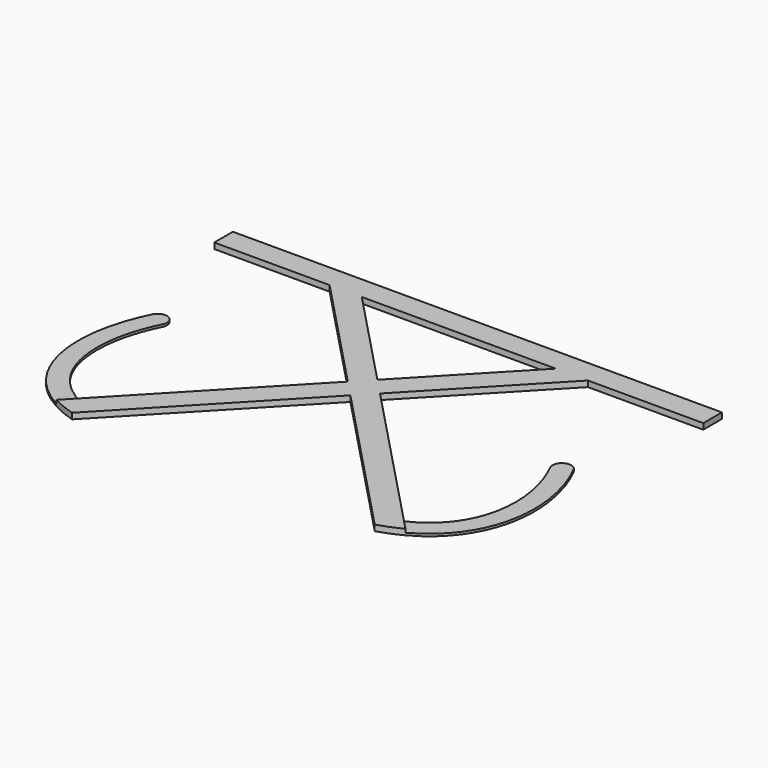
from build123d import *

# Parameters (mm, degrees)
F1_DEPTH = 2.5
F2_DEPTH = 1


with BuildPart() as f1:
    # F0 (on Top) → F1 (new body)
    with BuildSketch(Plane.XY):
        Polygon((51.1834802784, 68.1774026233), (-51.1834802784, 68.1774026233), (-41.6495295118, 58.1774026233), (41.6495295118, 58.1774026233), align=None)
        Polygon((55.4660492335, 58.1774026233), (41.6495295118, 58.1774026233), (0, 14.4919142756), (6.9082598608, 7.2459571378), align=None)
        Polygon((65, 68.1774026233), (51.1834802784, 68.1774026233), (41.6495295118, 58.1774026233), (55.4660492335, 58.1774026233), align=None)
        Polygon((105, 68.1774026233), (65, 68.1774026233), (55.4660492335, 58.1774026233), (105, 58.1774026233), align=None)
        Polygon((0, 14.4919142756), (-6.9082598608, 7.2459571378), (0, 0), (6.9082598608, 7.2459571378), align=None)
        Polygon((-41.6495295118, 58.1774026233), (-55.4660492335, 58.1774026233), (-6.9082598608, 7.2459571378), (0, 14.4919142756), align=None)
        Polygon((-65, 68.1774026233), (-105, 68.1774026233), (-105, 58.1774026233), (-55.4660492335, 58.1774026233), align=None)
        Polygon((-51.1834802784, 68.1774026233), (-65, 68.1774026233), (-55.4660492335, 58.1774026233), (-41.6495295118, 58.1774026233), align=None)
        Polygon((0, 0), (-6.9082598608, 7.2459571378), (-69.1652305646, -58.0543283665), (-72.2377126812, -61.2770029868), (-65, -68.1774026233), align=None)
        Polygon((6.9082598608, 7.2459571378), (0, 0), (65, -68.1774026233), (72.2377126812, -61.2770029868), (69.1652305646, -58.0543283665), align=None)
        with BuildLine():
            Line((72.2377126812, -61.2770029868), (65, -68.1774026233))
            add(Edge.make_bspline(
                [(65, -68.1774026233), (68.6268745658, -67.0893650818), (71.9339432438, -65.7183547634), (74.930951741, -64.1018959674)],
                knots=[0, 0, 0, 0, 8.3760284317, 8.3760284317, 8.3760284317, 8.3760284317], degree=3))
            Line((74.930951741, -64.1018959674), (72.2377126812, -61.2770029868))
        make_face()
        with BuildLine():
            add(Edge.make_bspline(
                [(-65, -68.1774026233), (-68.6268745658, -67.0893650818), (-71.9339432438, -65.7183547634), (-74.930951741, -64.1018959674)],
                knots=[0, 0, 0, 0, 8.3760284317, 8.3760284317, 8.3760284317, 8.3760284317], degree=3))
            Line((-65, -68.1774026233), (-72.2377126812, -61.2770029868))
            Line((-72.2377126812, -61.2770029868), (-74.930951741, -64.1018959674))
        make_face()
    extrude(amount=F1_DEPTH)

    # F0 (on Top) → F2 (join)
    with BuildSketch(Plane.XY):
        with BuildLine():
            Line((-72.2377126812, -61.2770029868), (-69.1652305646, -58.0543283665))
            add(Edge.make_bspline(
                [(-69.1652305646, -58.0543283665), (-70.3250835979, -57.5069886319), (-74.4014214589, -55.3435693139), (-80.1194434399, -50.8178129439), (-85.3002038596, -43.8525742273), (-88.6335778365, -35.7264574842), (-90.1326278523, -26.600736586), (-89.7619779119, -16.7792607957), (-87.522930234, -6.6468948829), (-84.8180719607, 0.043101538), (-83.1770195254, 3.3049470114)],
                knots=[0.078777441, 0.078777441, 0.078777441, 0.078777441, 0.125, 0.25, 0.375, 0.5, 0.625, 0.75, 0.875, 1, 1, 1, 1], degree=3))
            ThreePointArc((-83.1770195254, 3.3049470114), (-84.9983423891, 8.5849173617), (-90.3235375881, 6.9003996365))
            add(Edge.make_bspline(
                [(-74.930951741, -64.1018959674), (-100.2843329163, -50.4273614959), (-103.4485051858, -19.187502997), (-90.3235375881, 6.9003996365)],
                knots=[8.3760284317, 8.3760284317, 8.3760284317, 8.3760284317, 79.2335657922, 79.2335657922, 79.2335657922, 79.2335657922], degree=3))
            Line((-74.930951741, -64.1018959674), (-72.2377126812, -61.2770029868))
        make_face()
        with BuildLine():
            add(Edge.make_bspline(
                [(69.1652305646, -58.0543283665), (70.3250835979, -57.5069886319), (74.4014214589, -55.3435693139), (80.1194434399, -50.8178129439), (85.3002038596, -43.8525742273), (88.6335778365, -35.7264574842), (90.1326278523, -26.600736586), (89.7619779119, -16.7792607957), (87.522930234, -6.6468948829), (84.8180719607, 0.043101538), (83.1770195254, 3.3049470114)],
                knots=[0.078777441, 0.078777441, 0.078777441, 0.078777441, 0.125, 0.25, 0.375, 0.5, 0.625, 0.75, 0.875, 1, 1, 1, 1], degree=3))
            Line((69.1652305646, -58.0543283665), (72.2377126812, -61.2770029868))
            Line((72.2377126812, -61.2770029868), (74.930951741, -64.1018959674))
            add(Edge.make_bspline(
                [(74.930951741, -64.1018959674), (100.2843329163, -50.4273614959), (103.4485051858, -19.187502997), (90.3235375881, 6.9003996365)],
                knots=[8.3760284317, 8.3760284317, 8.3760284317, 8.3760284317, 79.2335657922, 79.2335657922, 79.2335657922, 79.2335657922], degree=3))
            ThreePointArc((90.3235375881, 6.9003996365), (84.9983423891, 8.5849173617), (83.1770195254, 3.3049470114))
        make_face()
    extrude(amount=F2_DEPTH)


solid = f1.part
